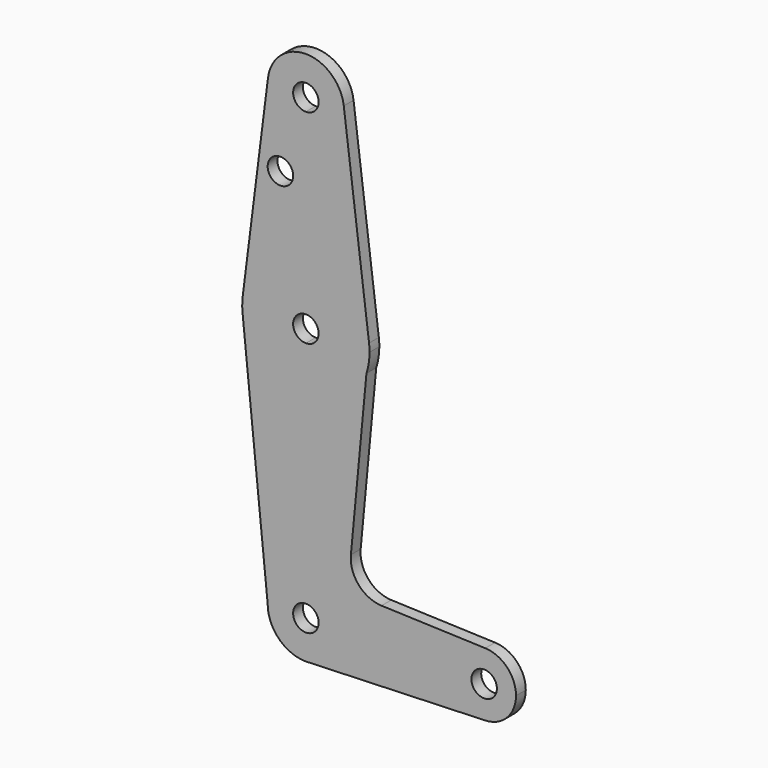
from build123d import *

# Parameters (mm, degrees)
F0_R     = 3.175
F1_DEPTH = 3.048


with BuildPart() as f1:
    # F0 (on Front) → F1 (new body)
    with BuildSketch(Plane.XZ):
        with BuildLine():
            ThreePointArc((3.175, 0), (-2.2450640303, -2.2450640303), (0, 3.175))
            Line((0, 3.175), (0, 9.525))
            ThreePointArc((0, 9.525), (-6.7351920908, 6.7351920908), (-9.525, 0))
            ThreePointArc((-9.525, 0), (-6.7351920908, -6.7351920908), (0, -9.525))
            Line((0, -9.525), (0.6773435479, -9.500885786))
            ThreePointArc((0.6773435479, -9.500885786), (6.9705567315, -6.4912990883), (9.525, 0))
            Line((9.525, 0), (3.175, 0))
        make_face()
        with BuildLine():
            Line((0, 9.525), (0, 3.175))
            ThreePointArc((0, 3.175), (2.2450640303, 2.2450640303), (3.175, 0))
            Line((3.175, 0), (9.525, 0))
            ThreePointArc((9.525, 0), (6.7351920908, 6.7351920908), (0, 9.525))
        make_face()
        with BuildLine():
            ThreePointArc((-9.525, 0), (-6.7351920908, 6.7351920908), (0, 9.525))
            Line((0, 9.525), (0, 47.625))
            ThreePointArc((0, 47.625), (-10.5003255158, 51.59375), (-15.7504882737, 61.515625))
            ThreePointArc((-15.7504882737, 61.515625), (-15.7735187252, 61.707869417), (-15.7942028036, 61.9003804205))
            Line((-15.7942028036, 61.9003804205), (-9.525, 0))
        make_face()
        with BuildLine():
            Line((0, 47.625), (0, 9.525))
            ThreePointArc((0, 9.525), (6.7351920908, 6.7351920908), (9.525, 0))
            Line((9.525, 0), (36.5125, 0))
            ThreePointArc((36.5125, 0), (38.9384772185, 5.7120069047), (44.7334821429, 7.9324362036))
            Line((44.7334821429, 7.9324362036), (18.8554927994, 8.8572400953))
            ThreePointArc((18.8554927994, 8.8572400953), (13.1648666795, 11.5573428462), (11.2244328628, 17.5497127533))
            Line((11.2244328628, 17.5497127533), (15.1007031189, 58.6026139305))
            ThreePointArc((15.1007031189, 58.6026139305), (9.3346028611, 50.6594075516), (0, 47.625))
        make_face()
        with BuildLine():
            Line((36.5125, 0), (9.525, 0))
            ThreePointArc((9.525, 0), (6.9705567315, -6.4912990883), (0.6773435479, -9.500885786))
            Line((0.6773435479, -9.500885786), (44.7324052746, -7.9324746146))
            ThreePointArc((44.7324052746, -7.9324746146), (38.9380895153, -5.7116327839), (36.5125, 0))
        make_face()
        with BuildLine():
            ThreePointArc((-15.7504882737, 61.515625), (-10.5003255158, 51.59375), (0, 47.625))
            Line((0, 47.625), (0, 60.325))
            ThreePointArc((0, 60.325), (-3.175, 63.5), (0, 66.675))
            Line((0, 66.675), (0, 79.375))
            ThreePointArc((0, 79.375), (-10.5003255158, 75.40625), (-15.7504882737, 65.484375))
            Line((-15.7504882737, 65.484375), (-15.7504882737, 61.515625))
        make_face()
        with BuildLine():
            Line((0, 60.325), (0, 47.625))
            ThreePointArc((0, 47.625), (9.3346028611, 50.6594075516), (15.1007031189, 58.6026139305))
            Line((15.1007031189, 58.6026139305), (15.7504882737, 65.484375))
            ThreePointArc((15.7504882737, 65.484375), (10.5003255158, 75.40625), (0, 79.375))
            Line((0, 79.375), (0, 66.675))
            ThreePointArc((0, 66.675), (2.2450640303, 65.7450640303), (3.175, 63.5))
            ThreePointArc((3.175, 63.5), (2.2450640303, 61.2549359697), (0, 60.325))
        make_face()
        with BuildLine():
            ThreePointArc((44.7334821429, 7.9324362036), (38.9384772185, 5.7120069047), (36.5125, 0))
            ThreePointArc((36.5125, 0), (38.9380895153, -5.7116327839), (44.7324052746, -7.9324746146))
            ThreePointArc((44.7324052746, -7.9324746146), (50.1616327839, -5.5119104847), (52.3875, 0))
            ThreePointArc((52.3875, 0), (50.1620069047, 5.5115227815), (44.7334821429, 7.9324362036))
        make_face()
        with BuildLine():
            ThreePointArc((47.625, 0), (44.45, -3.175), (41.275, 0))
            ThreePointArc((41.275, 0), (44.45, 3.175), (47.625, 0))
        make_face(mode=Mode.SUBTRACT)
        with BuildLine():
            ThreePointArc((0, -9.525), (0.3388863295, -9.5189695375), (0.6773435479, -9.500885786))
            Line((0.6773435479, -9.500885786), (0, -9.525))
        make_face()
        with BuildLine():
            ThreePointArc((-15.7942028036, 61.9003804205), (-15.7735187252, 61.707869417), (-15.7504882737, 61.515625))
            Line((-15.7504882737, 61.515625), (-15.7504882737, 65.484375))
            ThreePointArc((-15.7504882737, 65.484375), (-15.8738192656, 63.6936154008), (-15.7942028036, 61.9003804205))
        make_face()
        with BuildLine():
            Line((15.7504882737, 65.484375), (15.1007031189, 58.6026139305))
            ThreePointArc((15.1007031189, 58.6026139305), (15.6802309775, 61.020890988), (15.875, 63.5))
            ThreePointArc((15.875, 63.5), (15.8438414904, 64.4941387366), (15.7504882737, 65.484375))
        make_face()
        with BuildLine():
            Line((-9.4502929642, 115.490625), (-15.7504882737, 65.484375))
            ThreePointArc((-15.7504882737, 65.484375), (-10.5003255158, 75.40625), (0, 79.375))
            Line((0, 79.375), (0, 104.775))
            ThreePointArc((0, 104.775), (-7.14375, 107.9998046905), (-9.4502929642, 115.490625))
        make_face()
        with Locations((-6.35, 96.0330771523)):
            Circle(F0_R, mode=Mode.SUBTRACT)
        with BuildLine():
            ThreePointArc((0, 79.375), (10.5003255158, 75.40625), (15.7504882737, 65.484375))
            Line((15.7504882737, 65.484375), (9.4502929642, 115.490625))
            ThreePointArc((9.4502929642, 115.490625), (9.5063048942, 114.896483242), (9.525, 114.3))
            ThreePointArc((9.525, 114.3), (6.7351920908, 107.5648079092), (0, 104.775))
            Line((0, 104.775), (0, 79.375))
        make_face()
        with BuildLine():
            ThreePointArc((9.4502929642, 115.490625), (0, 123.825), (-9.4502929642, 115.490625))
            ThreePointArc((-9.4502929642, 115.490625), (-7.14375, 107.9998046905), (0, 104.775))
            ThreePointArc((0, 104.775), (6.7351920908, 107.5648079092), (9.525, 114.3))
            ThreePointArc((9.525, 114.3), (9.5063048942, 114.896483242), (9.4502929642, 115.490625))
        make_face()
        with BuildLine():
            ThreePointArc((3.175, 114.3), (2.2450640303, 112.0549359697), (0, 111.125))
            ThreePointArc((0, 111.125), (-2.2450640303, 116.5450640303), (3.175, 114.3))
        make_face(mode=Mode.SUBTRACT)
    extrude(amount=F1_DEPTH)


solid = f1.part
